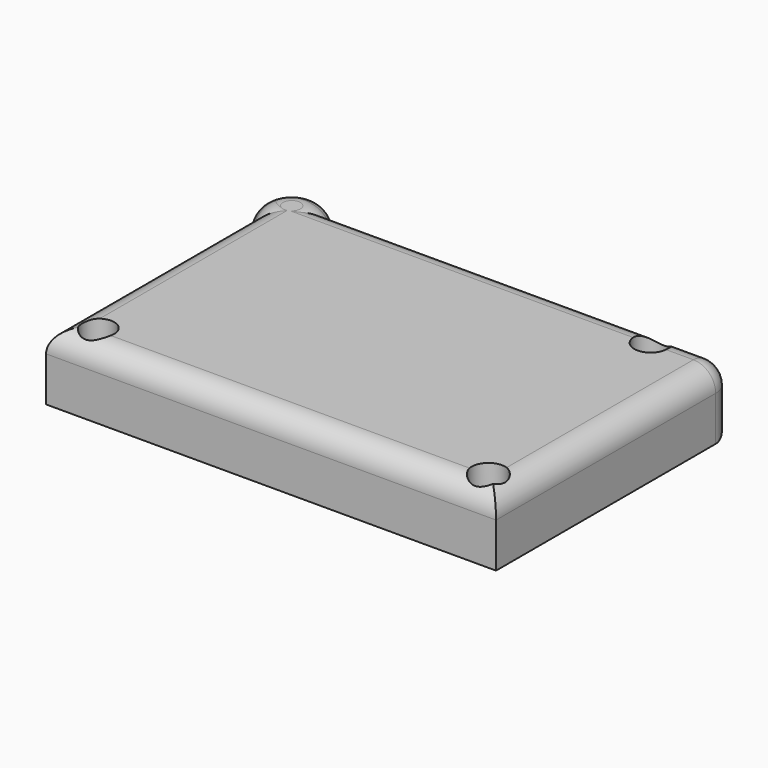
from build123d import *

# Parameters (mm, degrees)
F0_R         = 3.586786404
F0_R_2       = 3.7582992631
F0_R_3       = 3.6865102679
F1_DEPTH     = 15
F2_T1_DEPTH  = 126.0138504207
F2_T3_DEPTH  = 22.5
F2_T5_DEPTH  = 74.126155749
F2_S9_W      = 5
F2_S9_H      = 5
F2_T10_DEPTH = 5
F2_T16_DEPTH = 97.9066217834
F2_S17_R     = 6.9574459714
F2_T18_DEPTH = 51
F2_T22_DEPTH = 82.9931766736
F2_S23_R     = 6.9574459714
F2_T24_DEPTH = 43
F2_T28_ANGLE = 359.64
F2_T34_ANGLE = 359.64
F2_T40_ANGLE = 359.64
F2_T46_DEPTH = 115.4066217834
F2_S47_R     = 6.9574459714
F2_T48_DEPTH = 59
F2_T53_ANGLE = 359.64
F2_T58_DEPTH = 97.9066217834
F2_S59_R     = 6.9574459714
F2_T60_DEPTH = 51
F2_T66_ANGLE = 359.64
F2_T71_DEPTH = 82.9931766736
F2_S72_R     = 6.9574459714
F2_T73_DEPTH = 43


# Not quite as in the source:
# - a fillet or chamfer that OpenCascade refuses, or shapes differently, is made with other operations: its cross-section is extruded or revolved along the edge and cut away or added


with BuildPart() as f1:
    # F0 (on Top) → F1 (new body)
    with BuildSketch(Plane.XY):
        with BuildLine():
            Line((-47.5761555135, 22.2377919602), (-47.5761555135, 30.8707710356))
            Line((-47.5761555135, 30.8707710356), (-36.9689268762, 30.8707710356))
            ThreePointArc((-36.9689268762, 30.8707710356), (-47.4740962985, 32.9453643179), (-47.5761555135, 22.2377919602))
        make_face()
        with BuildLine():
            Line((-36.9689268762, 30.8707710356), (-47.5761555135, 30.8707710356))
            Line((-47.5761555135, 30.8707710356), (-47.5761555135, 22.2377919602))
            ThreePointArc((-47.5761555135, 22.2377919602), (-40.1548216165, 21.2376644422), (-36.1248620528, 27.5492314249))
            ThreePointArc((-36.1248620528, 27.5492314249), (-36.3391791701, 29.2627855393), (-36.9689268762, 30.8707710356))
        make_face()
        with BuildLine():
            Line((53.4376949072, 30.8707710356), (-36.9689268762, 30.8707710356))
            ThreePointArc((-36.9689268762, 30.8707710356), (-36.3391791701, 29.2627855393), (-36.1248620528, 27.5492314249))
            ThreePointArc((-36.1248620528, 27.5492314249), (-40.1548216165, 21.2376644422), (-47.5761555135, 22.2377919602))
            Line((-47.5761555135, 22.2377919602), (-47.5761555135, -35.7553847134))
            Line((-47.5761555135, -35.7553847134), (53.4376949072, -35.7553847134))
            Line((53.4376949072, -35.7553847134), (53.4376949072, 30.8707710356))
        make_face()
        with Locations((-40.5423082411, -29.8938471824)):
            Circle(F0_R, mode=Mode.SUBTRACT)
        with Locations((47.1853874624, -30.089231208)):
            Circle(F0_R_2, mode=Mode.SUBTRACT)
        with Locations((38.5884605348, 26.1815395206)):
            Circle(F0_R_3, mode=Mode.SUBTRACT)
    extrude(amount=F1_DEPTH)

    # F2: fillet of radius 5 on 7 edges, made by hand

    # F2_s2 → F2_t1 (cut)
    with BuildSketch(Plane.YZ.offset(-60.0761555135)):
        with BuildLine():
            ThreePointArc((-35.7553847134, 10), (-34.2909186193, 13.5355339059), (-30.7553847134, 15))
            Line((-30.7553847134, 15), (-35.7553847134, 15))
            Line((-35.7553847134, 15), (-35.7553847134, 10))
        make_face()
    extrude(amount=F2_T1_DEPTH, mode=Mode.SUBTRACT)

    # F2_s4 → F2_t3 (cut)
    with BuildSketch(Plane.XY.offset(-12.5)):
        with BuildLine():
            ThreePointArc((53.4376949072, 25.8707710356), (51.9732288131, 29.4063049415), (48.4376949072, 30.8707710356))
            Line((48.4376949072, 30.8707710356), (53.4376949072, 30.8707710356))
            Line((53.4376949072, 30.8707710356), (53.4376949072, 25.8707710356))
        make_face()
    extrude(amount=F2_T3_DEPTH, mode=Mode.SUBTRACT)

    # F2_s6 → F2_t5 (cut)
    with BuildSketch(Plane.XZ.offset(-25.8707710356)):
        with BuildLine():
            ThreePointArc((53.4376949072, 10), (51.9732288131, 13.5355339059), (48.4376949072, 15))
            Line((48.4376949072, 15), (53.4376949072, 15))
            Line((53.4376949072, 15), (53.4376949072, 10))
        make_face()
    extrude(amount=F2_T5_DEPTH, mode=Mode.SUBTRACT)


with BuildPart() as f2_tool8:
    # F2_s9 → F2_t10 (new body)
    with BuildSketch(Plane.XY.offset(10)):
        with Locations((50.9376949072, 28.3707710356)):
            Rectangle(F2_S9_W, F2_S9_H)
    extrude(amount=F2_T10_DEPTH)

    # F2_s11 → F2_t12 (revolve, cut)
    with BuildSketch(Plane(origin=(48.4376949072, 25.8707710356, 10), x_dir=(-0.7071067812, -0.7071067812, 0), z_dir=(-0.7071067812, 0.7071067812, 0))):
        with BuildLine():
            ThreePointArc((0, -5), (5, 0), (0, 5))
            Line((0, 5), (0, -5))
        make_face()
    revolve(axis=Axis((48.4376949072, 25.8707710356, 10), (0, 0, 1)), mode=Mode.SUBTRACT)


with BuildPart() as f1_1:
    add(f1.part)

    # F2_t7: cut F2_tool8
    add(f2_tool8.part, mode=Mode.SUBTRACT)


with BuildPart() as f2_tool14:
    # F2_s15 → F2_t16 (new body)
    with BuildSketch(Plane.YZ.offset(48.4376949072)):
        with BuildLine():
            ThreePointArc((30.8707710356, 10), (29.4063049415, 13.5355339059), (25.8707710356, 15))
            Line((25.8707710356, 15), (30.8707710356, 15))
            Line((30.8707710356, 15), (30.8707710356, 10))
        make_face()
    extrude(amount=-F2_T16_DEPTH)

    # F2_s17 → F2_t18 (cut, symmetric)
    with BuildSketch(Plane.XY.offset(12.5)):
        with Locations((-43.0823080242, 27.5492314249)):
            Circle(F2_S17_R)
    extrude(amount=F2_T18_DEPTH, both=True, mode=Mode.SUBTRACT)


with BuildPart() as f1_2:
    add(f1_1.part)

    # F2_t13: cut F2_tool14
    add(f2_tool14.part, mode=Mode.SUBTRACT)


with BuildPart() as f2_tool20:
    # F2_s21 → F2_t22 (new body)
    with BuildSketch(Plane.XZ.offset(-34.7377919602)):
        with BuildLine():
            ThreePointArc((-47.5761555135, 10), (-46.1116894195, 13.5355339059), (-42.5761555135, 15))
            Line((-42.5761555135, 15), (-47.5761555135, 15))
            Line((-47.5761555135, 15), (-47.5761555135, 10))
        make_face()
    extrude(amount=F2_T22_DEPTH)

    # F2_s23 → F2_t24 (cut, symmetric)
    with BuildSketch(Plane.XY.offset(12.5)):
        with Locations((-43.0823080242, 27.5492314249)):
            Circle(F2_S23_R)
    extrude(amount=F2_T24_DEPTH, both=True, mode=Mode.SUBTRACT)


with BuildPart() as f1_3:
    add(f1_2.part)

    # F2_t19: cut F2_tool20
    add(f2_tool20.part, mode=Mode.SUBTRACT)


with BuildPart() as f2_tool26:
    # F2_s27 → F2_t28 (revolve)
    with BuildSketch(Plane(origin=(-12.2782997509, -10.0573142374, 0), x_dir=(0, 0, 1), z_dir=(-0.77360415, -0.6336691716, 0))):
        with BuildLine():
            ThreePointArc((10, 41.6546842262), (13.5355339059, 43.1191503203), (15, 46.6546842262))
            Line((15, 46.6546842262), (15, 41.6546842262))
            Line((15, 41.6546842262), (10, 41.6546842262))
        make_face()
    revolve(axis=Axis((-43.0823080242, 27.5492314249, 15), (0, 0, 1)), revolution_arc=F2_T28_ANGLE)

    split(bisect_by=Plane.XZ.offset(-30.8707710356), keep=Keep.TOP)

    split(bisect_by=Plane.YZ.offset(-47.5761555135), keep=Keep.BOTTOM)


with BuildPart() as f1_4:
    add(f1_3.part)

    # F2_t25: cut F2_tool26
    add(f2_tool26.part, mode=Mode.SUBTRACT)


with BuildPart() as f2_tool32:
    # F2_s33 → F2_t34 (revolve)
    with BuildSketch(Plane(origin=(-12.2782997509, -10.0573142374, 0), x_dir=(0, 0, 1), z_dir=(-0.77360415, -0.6336691716, 0))):
        with BuildLine():
            ThreePointArc((10, 41.6546842262), (13.5355339059, 43.1191503203), (15, 46.6546842262))
            Line((15, 46.6546842262), (15, 41.6546842262))
            Line((15, 41.6546842262), (10, 41.6546842262))
        make_face()
    revolve(axis=Axis((-43.0823080242, 27.5492314249, 15), (0, 0, 1)), revolution_arc=F2_T34_ANGLE)

    split(bisect_by=Plane.XZ.offset(-30.8707710356), keep=Keep.BOTTOM)

    split(bisect_by=Plane.YZ.offset(-47.5761555135), keep=Keep.TOP)


with BuildPart() as f1_5:
    add(f1_4.part)

    # F2_t31: cut F2_tool32
    add(f2_tool32.part, mode=Mode.SUBTRACT)


with BuildPart() as f2_tool38:
    # F2_s39 → F2_t40 (revolve)
    with BuildSketch(Plane(origin=(-12.2782997509, -10.0573142374, 0), x_dir=(0, 0, 1), z_dir=(-0.77360415, -0.6336691716, 0))):
        with BuildLine():
            ThreePointArc((10, 41.6546842262), (13.5355339059, 43.1191503203), (15, 46.6546842262))
            Line((15, 46.6546842262), (15, 41.6546842262))
            Line((15, 41.6546842262), (10, 41.6546842262))
        make_face()
    revolve(axis=Axis((-43.0823080242, 27.5492314249, 15), (0, 0, 1)), revolution_arc=F2_T40_ANGLE)

    split(bisect_by=Plane.XZ.offset(-30.8707710356), keep=Keep.BOTTOM)

    split(bisect_by=Plane.YZ.offset(-47.5761555135), keep=Keep.BOTTOM)


with BuildPart() as f1_6:
    add(f1_5.part)

    # F2_t37: cut F2_tool38
    add(f2_tool38.part, mode=Mode.SUBTRACT)


with BuildPart() as f2_tool44:
    # F2_s45 → F2_t46 (new body)
    with BuildSketch(Plane.YZ.offset(65.9376949072)):
        with BuildLine():
            ThreePointArc((30.8707710356, 5), (29.4063049415, 1.4644660941), (25.8707710356, 0))
            Line((25.8707710356, 0), (30.8707710356, 0))
            Line((30.8707710356, 0), (30.8707710356, 5))
        make_face()
    extrude(amount=-F2_T46_DEPTH)

    # F2_s47 → F2_t48 (cut, symmetric)
    with BuildSketch(Plane.XY.offset(2.5)):
        with Locations((-43.0823080242, 27.5492314249)):
            Circle(F2_S47_R)
    extrude(amount=F2_T48_DEPTH, both=True, mode=Mode.SUBTRACT)


with BuildPart() as f1_7:
    add(f1_6.part)

    # F2_t43: cut F2_tool44
    add(f2_tool44.part, mode=Mode.SUBTRACT)


with BuildPart() as f2_tool51:
    # F2_s52 → F2_t53 (revolve)
    with BuildSketch(Plane(origin=(-12.2782997509, -10.0573142374, 0), x_dir=(0, 0, 1), z_dir=(-0.77360415, -0.6336691716, 0))):
        with BuildLine():
            ThreePointArc((10, 41.6546842262), (13.5355339059, 43.1191503203), (15, 46.6546842262))
            Line((15, 46.6546842262), (15, 41.6546842262))
            Line((15, 41.6546842262), (10, 41.6546842262))
        make_face()
    revolve(axis=Axis((-43.0823080242, 27.5492314249, 15), (0, 0, 1)), revolution_arc=F2_T53_ANGLE)

    split(bisect_by=Plane.XZ.offset(-30.8707710356), keep=Keep.TOP)

    split(bisect_by=Plane.YZ.offset(-47.5761555135), keep=Keep.TOP)


with BuildPart() as f2_tool56:
    # F2_s57 → F2_t58 (new body)
    with BuildSketch(Plane.YZ.offset(48.4376949072)):
        with BuildLine():
            ThreePointArc((30.8707710356, 10), (29.4063049415, 13.5355339059), (25.8707710356, 15))
            Line((25.8707710356, 15), (30.8707710356, 15))
            Line((30.8707710356, 15), (30.8707710356, 10))
        make_face()
    extrude(amount=-F2_T58_DEPTH)

    # F2_s59 → F2_t60 (intersect, symmetric)
    with BuildSketch(Plane.XY.offset(12.5)):
        with Locations((-43.0823080242, 27.5492314249)):
            Circle(F2_S59_R)
    extrude(amount=F2_T60_DEPTH, both=True, mode=Mode.INTERSECT)


with BuildPart() as f2_tool51_1:
    add(f2_tool51.part)

    # F2_t61: intersect F2_tool56
    add(f2_tool56.part, mode=Mode.INTERSECT)


with BuildPart() as f1_8:
    add(f1_7.part)

    # F2_t49: cut F2_tool51
    add(f2_tool51_1.part, mode=Mode.SUBTRACT)


with BuildPart() as f2_tool64:
    # F2_s65 → F2_t66 (revolve)
    with BuildSketch(Plane(origin=(-12.2782997509, -10.0573142374, 0), x_dir=(0, 0, 1), z_dir=(-0.77360415, -0.6336691716, 0))):
        with BuildLine():
            ThreePointArc((10, 41.6546842262), (13.5355339059, 43.1191503203), (15, 46.6546842262))
            Line((15, 46.6546842262), (15, 41.6546842262))
            Line((15, 41.6546842262), (10, 41.6546842262))
        make_face()
    revolve(axis=Axis((-43.0823080242, 27.5492314249, 15), (0, 0, 1)), revolution_arc=F2_T66_ANGLE)

    split(bisect_by=Plane.XZ.offset(-30.8707710356), keep=Keep.TOP)

    split(bisect_by=Plane.YZ.offset(-47.5761555135), keep=Keep.TOP)


with BuildPart() as f2_tool69:
    # F2_s70 → F2_t71 (new body)
    with BuildSketch(Plane.XZ.offset(-34.7377919602)):
        with BuildLine():
            ThreePointArc((-47.5761555135, 10), (-46.1116894195, 13.5355339059), (-42.5761555135, 15))
            Line((-42.5761555135, 15), (-47.5761555135, 15))
            Line((-47.5761555135, 15), (-47.5761555135, 10))
        make_face()
    extrude(amount=F2_T71_DEPTH)

    # F2_s72 → F2_t73 (intersect, symmetric)
    with BuildSketch(Plane.XY.offset(12.5)):
        with Locations((-43.0823080242, 27.5492314249)):
            Circle(F2_S72_R)
    extrude(amount=F2_T73_DEPTH, both=True, mode=Mode.INTERSECT)


with BuildPart() as f2_tool64_1:
    add(f2_tool64.part)

    # F2_t74: intersect F2_tool69
    add(f2_tool69.part, mode=Mode.INTERSECT)


with BuildPart() as f1_9:
    add(f1_8.part)

    # F2_t62: cut F2_tool64
    add(f2_tool64_1.part, mode=Mode.SUBTRACT)


solid = f1_9.part
